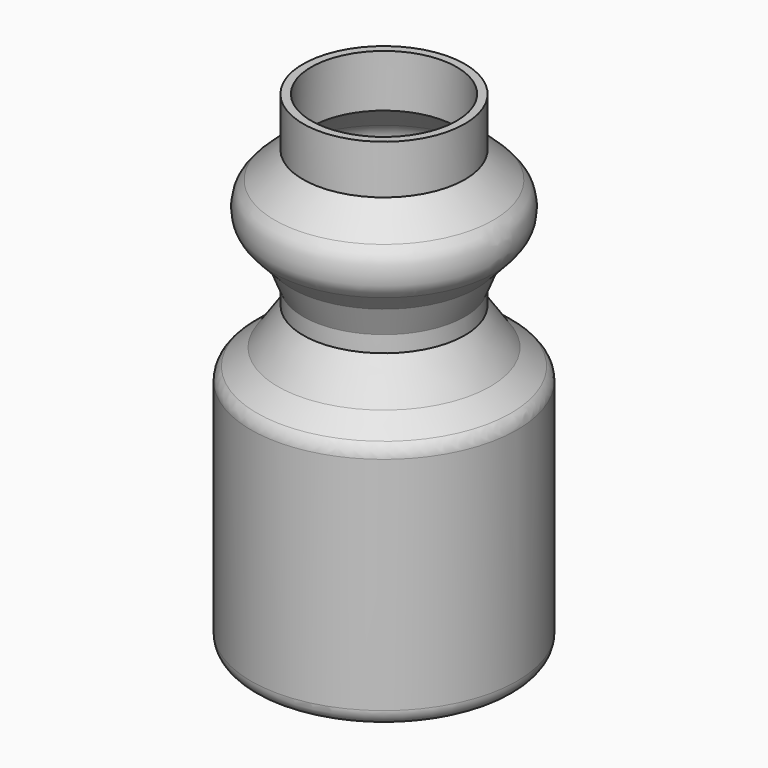
from build123d import *

# Parameters (mm, degrees)
F2_R    = 5
F3_R    = 10
F4_SIZE = 5
F5_R    = 5
F6_T    = -2.5


# Not quite as in the source:
# - a fillet or chamfer that OpenCascade refuses, or shapes differently, is made with other operations: its cross-section is extruded or revolved along the edge and cut away or added


with BuildPart() as f1:
    # F0 (on Front) → F1 (revolve)
    with BuildSketch(Plane.XZ):
        Polygon((0, 150), (0, 0), (40.7360860733, 0), (40.7360860733, 75.1049241643), (24.7445367592, 87.9864128578), (24.7445367592, 102.9864128578), (40.7360860733, 120), (24.7774192725, 135), (24.7774192725, 150), align=None)
    revolve(axis=Axis((0, 0, 75), (0, 0, -1)))

    # F2
    f2_edges = [f1.edges().sort_by_distance(p)[0] for p in [
        (-40.736086, 0, 0),
    ]]
    fillet(f2_edges, radius=F2_R)

    # F3
    f3_edges = [f1.edges().sort_by_distance(p)[0] for p in [
        (-40.736086, 0, 120),
    ]]
    fillet(f3_edges, radius=F3_R)

    # F4
    f4_edges = [f1.edges().sort_by_distance(p)[0] for p in [
        (-24.744537, 0, 102.986413),
    ]]
    chamfer(f4_edges, length=F4_SIZE)

    # F5
    f5_edges = [f1.edges().sort_by_distance(p)[0] for p in [
        (-40.736086, 0, 75.104924),
    ]]
    fillet(f5_edges, radius=F5_R)

    # F6
    f6_openings = [f1.faces().sort_by_distance(p)[0] for p in [
        (0, 0, 150),
    ]]
    offset(amount=F6_T, openings=f6_openings, kind=Kind.INTERSECTION)

    # F7: chamfer of 5 x 10 on 1 edges, made by hand

    # F7_s1 → F7_t2 (revolve)
    with BuildSketch(Plane.XZ):
        Polygon((32.5322168572, 81.7132925265), (24.7445367592, 92.9864128578), (24.7445367592, 87.9864128578), align=None)
    revolve(axis=Axis((0, 0, 87.9864128578), (0, 0, -1)))


solid = f1.part
